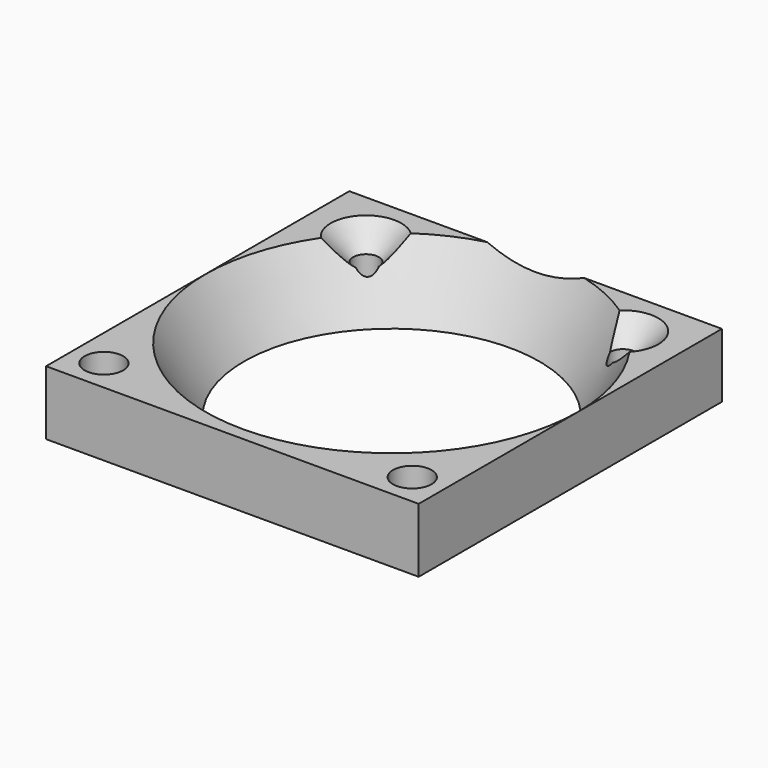
from build123d import *

# Parameters (mm, degrees)
F0_W        = 29
F0_H        = 29.5
F0_R        = 1.5
F0_R_2      = 1
F0_R_3      = 11.5
F1_DEPTH    = 5
F4_T2_ANGLE = 359.64
F4_T4_ANGLE = 359.64
F4_T6_ANGLE = 359.64


# Not quite as in the source:
# - a fillet or chamfer that OpenCascade refuses, or shapes differently, is made with other operations: its cross-section is extruded or revolved along the edge and cut away or added


with BuildPart() as f1:
    # F0 (on Top) → F1 (new body)
    with BuildSketch(Plane.XY):
        with Locations((0, -0.75)):
            Rectangle(F0_W, F0_H)
        with Locations((-12, -13)):
            Circle(F0_R, mode=Mode.SUBTRACT)
        with Locations((12, -13)):
            Circle(F0_R, mode=Mode.SUBTRACT)
        with Locations((-10, 10)):
            Circle(F0_R_2, mode=Mode.SUBTRACT)
        Circle(F0_R_3, mode=Mode.SUBTRACT)
        with Locations((10, 10)):
            Circle(F0_R_2, mode=Mode.SUBTRACT)
    extrude(amount=F1_DEPTH)

    # F2 (on Right) → F3 (revolve, cut)
    with BuildSketch(Plane.YZ):
        Polygon((-14.5, 5), (-11.5, 0), (-11.5, 5), align=None)
    revolve(axis=Axis((0, 0, 6.3592060469), (0, 0, 1)), mode=Mode.SUBTRACT)

    # F4: chamfer of 1.75 on 3 edges, made by hand

    # F4_s1 → F4_t2 (revolve, cut)
    with BuildSketch(Plane(origin=(0.0313170241, 0.0315144155, 0), x_dir=(0, 0, 1), z_dir=(-0.7048818539, -0.7093247296, 0))):
        Polygon((3.25, 13.1420658351), (5, 11.3920658351), (5, 13.1420658351), align=None)
    revolve(axis=Axis((-10, 10, 5), (0, 0, 1)), revolution_arc=F4_T2_ANGLE, mode=Mode.SUBTRACT)

    # F4_s3 → F4_t4 (revolve, cut)
    with BuildSketch(Plane(origin=(-0.0624354204, 9.9367750216, 0), x_dir=(0, 0, 1), z_dir=(0.006283144, -0.9999802609, 0))):
        Polygon((5, -12.8126340482), (3.25, -11.0626340482), (5, -11.0626340482), align=None)
    revolve(axis=Axis((10, 10, 5), (0, 0, 1)), revolution_arc=F4_T4_ANGLE, mode=Mode.SUBTRACT)

    # F4_s5 → F4_t6 (revolve, cut)
    with BuildSketch(Plane.XZ.offset(-10)):
        Polygon((12.75, 5), (11, 3.25), (11, 5), align=None)
    revolve(axis=Axis((10, 10, 5), (0, 0, 1)), revolution_arc=F4_T6_ANGLE, mode=Mode.SUBTRACT)


solid = f1.part
